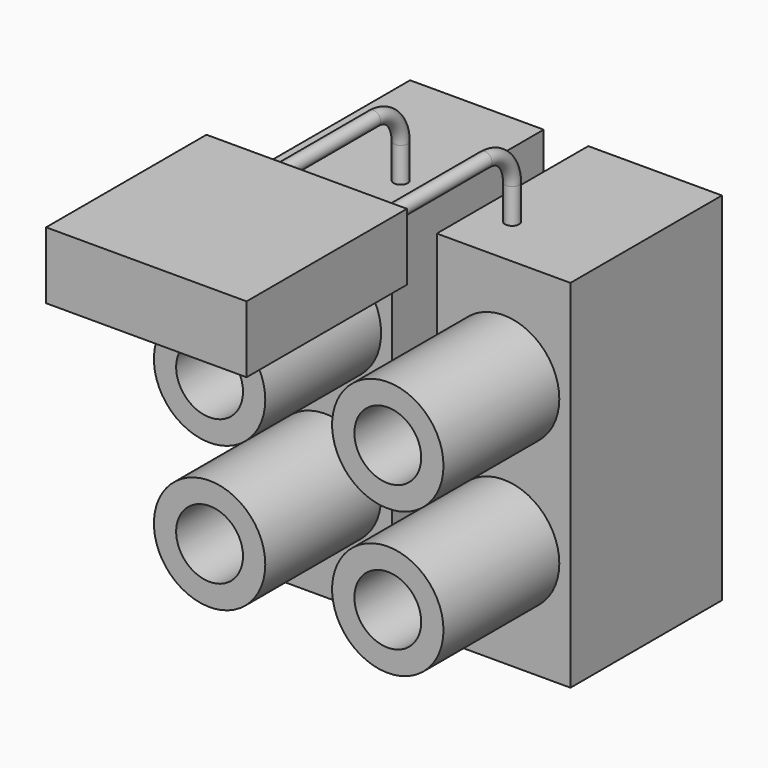
from build123d import *

# Parameters (mm, degrees)
F0_R     = 1.4
F1_DEPTH = 8.5
F2_R     = 2.5
F2_R_2   = 1.5
F3_DEPTH = 6.5
F5_W     = 9
F5_H     = 9
F6_DEPTH = 3
F9_R     = 0.3175


# Not quite as in the source:
# - a pattern or mirror of a feature is missing from the dataset's text; its kind, count and spacing are read off the source's solid


with BuildPart() as f1:
    # F0 (on Front) → F1 (new body)
    with BuildSketch(Plane.XZ):
        Polygon((-1, 8), (-7, 8), (-7, -8), (-1, -8), (-1, -1.75), (1, -1.75), (1, -8), (7, -8), (7, 8), (1, 8), (1, 1.75), (-1, 1.75), align=None)
        Circle(F0_R, mode=Mode.SUBTRACT)
    extrude(amount=F1_DEPTH)

    # F2 (on face) → F3 (join)
    with BuildSketch(Plane.XZ.offset(8.5)):
        with Locations((-4, 3.25)):
            Circle(F2_R)
        with Locations((-4, 3.25)):
            Circle(F2_R_2, mode=Mode.SUBTRACT)
        with Locations((-4, -3.25)):
            Circle(F2_R)
        with Locations((-4, -3.25)):
            Circle(F2_R_2, mode=Mode.SUBTRACT)
        with Locations((4, 3.25)):
            Circle(F2_R)
        with Locations((4, 3.25)):
            Circle(F2_R_2, mode=Mode.SUBTRACT)
        with Locations((4, -3.25)):
            Circle(F2_R)
        with Locations((4, -3.25)):
            Circle(F2_R_2, mode=Mode.SUBTRACT)
    extrude(amount=F3_DEPTH)


with BuildPart() as f6:
    # F5 (on offset) → F6 (new body)
    with BuildSketch(Plane.XY.offset(9.5748)):
        with Locations((0, -19.05)):
            Rectangle(F5_W, F5_H)
    extrude(amount=F6_DEPTH)

    # F10: sweep along a path in F8
    with BuildLine(Plane.YZ.offset(2.5)) as f10_path:
        Line((-14.55, 11.0748), (-7.675, 11.0748))
        ThreePointArc((-7.675, 11.0748), (-6.5973692655, 10.6284307345), (-6.151, 9.5508))
        Line((-6.151, 9.5508), (-6.151, 7.976))
    # F9 (on face) → F10 (sweep)
    with BuildSketch(Plane(origin=(0, -14.55, 0), x_dir=(-1, 0, 0), z_dir=(0, 1, 0))):
        with Locations((-2.5, 11.0748)):
            Circle(F9_R)
    f10 = sweep(path=f10_path.line)

    # F10_copies: F10 across plane
    add(f10.mirror(Plane(origin=(0, 0, 0), x_dir=(0, 0, -1), z_dir=(-1, 0, 0))))


solid = Compound([f1.part, f6.part])
